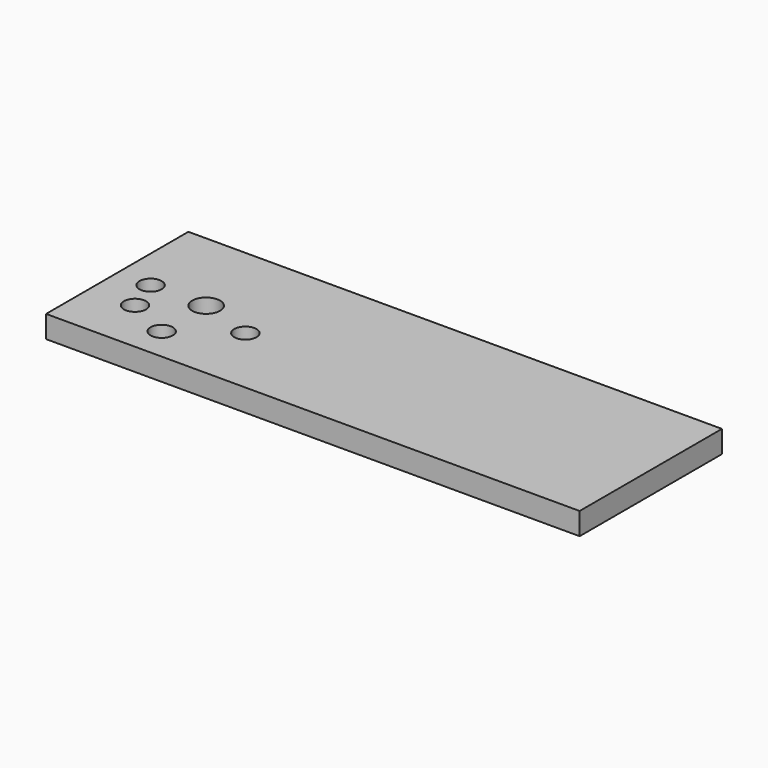
from build123d import *

# Parameters (mm, degrees)
F0_R     = 1.27
F1_DEPTH = 12.7
F3_D     = 15.875
F6_D     = 12.7
F8_D     = 12.7


# Not quite as in the source:
# - a feature names something its author has since deleted; it is built from what else it names


with BuildPart() as f1:
    # F0 (on Top) → F1 (new body)
    with BuildSketch(Plane.XY):
        Polygon((200.6098739386, 63.1592117809), (-2.5901260614, 63.1592117809), (-104.1901260614, 63.1592117809), (-104.1901260614, -38.4407882191), (-2.5901260614, -38.4407882191), (200.6098739386, -38.4407882191), align=None)
        with Locations((-53.3901260614, -19.3907882191)):
            Circle(F0_R, mode=Mode.SUBTRACT)
        with Locations((-78.4163327398, -7.1792497576)):
            Circle(F0_R, mode=Mode.SUBTRACT)
        with Locations((-53.3901260614, 12.3592117809)):
            Circle(F0_R, mode=Mode.SUBTRACT)
        with Locations((-23.1804483045, 2.5899810116)):
            Circle(F0_R, mode=Mode.SUBTRACT)
        with Locations((-85.1401260614, 12.3592117809)):
            Circle(F0_R, mode=Mode.SUBTRACT)
        with Locations((-92.6627071454, 25.0592117809)):
            Circle(F0_R, mode=Mode.SUBTRACT)
        with Locations((-12.1151260614, 12.3592117809)):
            Circle(F0_R, mode=Mode.SUBTRACT)
        with Locations((-20.8560573795, 37.7592117809)):
            Circle(F0_R, mode=Mode.SUBTRACT)
        with Locations((-53.3901260614, 53.6342117809)):
            Circle(F0_R, mode=Mode.SUBTRACT)
        with Locations((-92.6627071454, 25.0592117809)):
            Circle(F0_R)
        with Locations((-53.3901260614, 53.6342117809)):
            Circle(F0_R)
        with Locations((-20.8560573795, 37.7592117809)):
            Circle(F0_R)
        with Locations((-12.1151260614, 12.3592117809)):
            Circle(F0_R)
    extrude(amount=F1_DEPTH)

    # F3 (through all)
    with Locations(Plane.XY.offset(12.7)):
        with Locations((-53.3901260614, 12.3592117809)):
            Hole(F3_D / 2)

    # F6 (through all)
    with Locations(Plane.XY.offset(12.7)):
        with Locations((-53.3901260614, -19.3907882191)):
            Hole(F6_D / 2)

    # F8 (through all)
    with Locations(Plane.XY.offset(12.7)):
        with Locations((-85.1401260614, 12.3592117809), (-78.4163327398, -7.1792497576), (-23.1804483045, 2.5899810116)):
            Hole(F8_D / 2)


solid = f1.part
